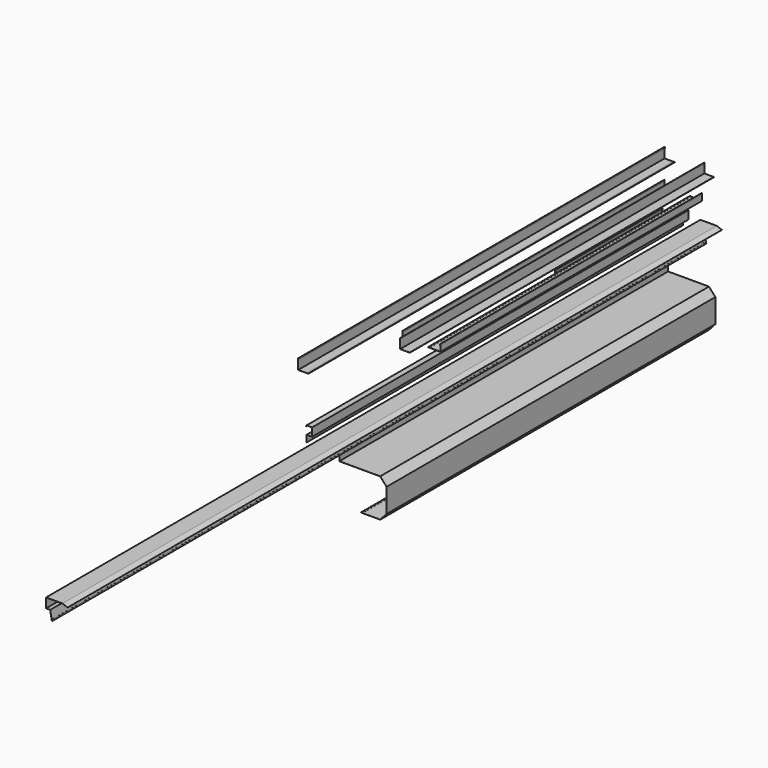
from build123d import *

# Parameters (mm, degrees)
F1_DEPTH  = 3360
F3_DEPTH  = 2790
F5_DEPTH  = 2400
F7_DEPTH  = 2400
F9_DEPTH  = 980
F11_DEPTH = 3450
F13_DEPTH = 6000
F15_DEPTH = 3015


# Not quite as in the source:
# - ends of sketch curves that miss each other by under 0.0002 mm in the source are joined


with BuildPart() as f1:
    # F0 (on Front) → F1 (new body)
    with BuildSketch(Plane.XZ):
        with BuildLine():
            Line((0, -75), (0, -0.5))
            ThreePointArc((0, -0.5), (0.1464466094, -0.1464466094), (0.5, 0))
            ThreePointArc((0.5, 0), (0.8535533906, -0.1464466094), (1, -0.5))
            Line((1, -0.5), (1, -10))
            Line((1, -10), (1.5, -10))
            Line((1.5, -10), (1.5, -0.5))
            ThreePointArc((1.5, -0.5), (1.2071067812, 0.2071067812), (0.5, 0.5))
            ThreePointArc((0.5, 0.5), (-0.2071067812, 0.2071067812), (-0.5, -0.5))
            Line((-0.5, -0.5), (-0.5, -75.5))
            Line((-0.5, -75.5), (74.5, -75.5))
            ThreePointArc((74.5, -75.5), (75.2071067812, -75.2071067812), (75.5, -74.5))
            ThreePointArc((75.5, -74.5), (75.2071067812, -73.7928932188), (74.5, -73.5))
            Line((74.5, -73.5), (65, -73.5))
            Line((65, -73.5), (65, -74))
            Line((65, -74), (74.5, -74))
            ThreePointArc((74.5, -74), (74.8535533906, -74.1464466094), (75, -74.5))
            ThreePointArc((75, -74.5), (74.8535533906, -74.8535533906), (74.5, -75))
            Line((74.5, -75), (0, -75))
        make_face()
    extrude(amount=F1_DEPTH)


with BuildPart() as f3:
    # F2 (on Front) → F3 (new body)
    with BuildSketch(Plane.XZ):
        with BuildLine():
            Line((291.6689515114, -7.9969086051), (291.6689515114, -77.4969086051))
            Line((291.6689515114, -77.4969086051), (361.1689515114, -77.4969086051))
            ThreePointArc((361.1689515114, -77.4969086051), (361.522504902, -77.6433552145), (361.6689515114, -77.9969086051))
            ThreePointArc((361.6689515114, -77.9969086051), (361.522504902, -78.3504619957), (361.1689515114, -78.4969086051))
            Line((361.1689515114, -78.4969086051), (351.6689515114, -78.4969086051))
            Line((351.6689515114, -78.4969086051), (351.6689515114, -78.9969086051))
            Line((351.6689515114, -78.9969086051), (361.1689515114, -78.9969086051))
            ThreePointArc((361.1689515114, -78.9969086051), (361.8760582926, -78.7040153863), (362.1689515114, -77.9969086051))
            ThreePointArc((362.1689515114, -77.9969086051), (361.8760582926, -77.2898018239), (361.1689515114, -76.9969086051))
            Line((361.1689515114, -76.9969086051), (292.1689515114, -76.9969086051))
            Line((292.1689515114, -76.9969086051), (292.1689515114, -7.9969086051))
            ThreePointArc((292.1689515114, -7.9969086051), (291.8760582926, -7.2898018239), (291.1689515114, -6.9969086051))
            ThreePointArc((291.1689515114, -6.9969086051), (290.4618447302, -7.2898018239), (290.1689515114, -7.9969086051))
            Line((290.1689515114, -7.9969086051), (290.1689515114, -17.4969086051))
            Line((290.1689515114, -17.4969086051), (290.6689515114, -17.4969086051))
            Line((290.6689515114, -17.4969086051), (290.6689515114, -7.9969086051))
            ThreePointArc((290.6689515114, -7.9969086051), (290.8153981208, -7.6433552145), (291.1689515114, -7.4969086051))
            ThreePointArc((291.1689515114, -7.4969086051), (291.522504902, -7.6433552145), (291.6689515114, -7.9969086051))
        make_face()
    extrude(amount=F3_DEPTH)


with BuildPart() as f5:
    # F4 (on Front) → F5 (new body)
    with BuildSketch(Plane.XZ):
        with BuildLine():
            Line((0, -212.6881961823), (0, -222.1881961823))
            Line((0, -222.1881961823), (0.5, -222.1881961823))
            Line((0.5, -222.1881961823), (0.5, -212.6881961823))
            ThreePointArc((0.5, -212.6881961823), (0.2071067812, -211.9810894011), (-0.5, -211.6881961823))
            ThreePointArc((-0.5, -211.6881961823), (-1.2071067812, -211.9810894011), (-1.5, -212.6881961823))
            Line((-1.5, -212.6881961823), (-1.5, -262.6881961823))
            Line((-1.5, -262.6881961823), (99.5, -262.6881961823))
            Line((99.5, -262.6881961823), (99.5, -212.6881961823))
            ThreePointArc((99.5, -212.6881961823), (99.2071067812, -211.9810894011), (98.5, -211.6881961823))
            ThreePointArc((98.5, -211.6881961823), (97.7928932188, -211.9810894011), (97.5, -212.6881961823))
            Line((97.5, -212.6881961823), (97.5, -222.1881961823))
            Line((97.5, -222.1881961823), (98, -222.1881961823))
            Line((98, -222.1881961823), (98, -212.6881961823))
            ThreePointArc((98, -212.6881961823), (98.1464466094, -212.3346427917), (98.5, -212.1881961823))
            ThreePointArc((98.5, -212.1881961823), (98.8535533906, -212.3346427917), (99, -212.6881961823))
            Line((99, -212.6881961823), (99, -262.1881961823))
            Line((99, -262.1881961823), (-1, -262.1881961823))
            Line((-1, -262.1881961823), (-1, -212.6881961823))
            ThreePointArc((-1, -212.6881961823), (-0.8535533906, -212.3346427917), (-0.5, -212.1881961823))
            ThreePointArc((-0.5, -212.1881961823), (-0.1464466094, -212.3346427917), (0, -212.6881961823))
        make_face()
    extrude(amount=F5_DEPTH)


with BuildPart() as f7:
    # F6 (on Front) → F7 (new body)
    with BuildSketch(Plane.XZ):
        with BuildLine():
            Line((186.1295764446, -256.9942643642), (195.6295764446, -256.9942643642))
            Line((195.6295764446, -256.9942643642), (195.6295764446, -256.4942643642))
            Line((195.6295764446, -256.4942643642), (186.1295764446, -256.4942643642))
            ThreePointArc((186.1295764446, -256.4942643642), (185.4224696634, -256.7871575831), (185.1295764446, -257.4942643642))
            ThreePointArc((185.1295764446, -257.4942643642), (185.4224696634, -258.2013711454), (186.1295764446, -258.4942643642))
            Line((186.1295764446, -258.4942643642), (276.1295764446, -258.4942643642))
            Line((276.1295764446, -258.4942643642), (276.1295764446, -208.4942643642))
            ThreePointArc((276.1295764446, -208.4942643642), (275.8366832258, -207.7871575831), (275.1295764446, -207.4942643642))
            ThreePointArc((275.1295764446, -207.4942643642), (274.4224696634, -207.7871575831), (274.1295764446, -208.4942643642))
            Line((274.1295764446, -208.4942643642), (274.1295764446, -217.9942643642))
            Line((274.1295764446, -217.9942643642), (274.6295764446, -217.9942643642))
            Line((274.6295764446, -217.9942643642), (274.6295764446, -208.4942643642))
            ThreePointArc((274.6295764446, -208.4942643642), (274.776023054, -208.1407109736), (275.1295764446, -207.9942643642))
            ThreePointArc((275.1295764446, -207.9942643642), (275.4831298352, -208.1407109736), (275.6295764446, -208.4942643642))
            Line((275.6295764446, -208.4942643642), (275.6295764446, -257.9942643642))
            Line((275.6295764446, -257.9942643642), (186.1295764446, -257.9942643642))
            ThreePointArc((186.1295764446, -257.9942643642), (185.776023054, -257.8478177548), (185.6295764446, -257.4942643642))
            ThreePointArc((185.6295764446, -257.4942643642), (185.776023054, -257.1407109736), (186.1295764446, -256.9942643642))
        make_face()
    extrude(amount=F7_DEPTH)


with BuildPart() as f9:
    # F8 (on Front) → F9 (new body)
    with BuildSketch(Plane.XZ):
        with BuildLine():
            Line((-18.0000039637, -452.1825845242), (-18.0000039637, -402.6825845242))
            ThreePointArc((-18.0000039637, -402.6825845242), (-17.8535573543, -402.3290311336), (-17.5000039637, -402.1825845242))
            ThreePointArc((-17.5000039637, -402.1825845242), (-17.1464505731, -402.3290311336), (-17.0000039637, -402.6825845242))
            Line((-17.0000039637, -402.6825845242), (-17.0000039637, -412.1825845242))
            Line((-17.0000039637, -412.1825845242), (-16.5000039637, -412.1825845242))
            Line((-16.5000039637, -412.1825845242), (-16.5000039637, -402.6825845242))
            ThreePointArc((-16.5000039637, -402.6825845242), (-16.7928971825, -401.975477743), (-17.5000039637, -401.6825845242))
            ThreePointArc((-17.5000039637, -401.6825845242), (-18.2071107449, -401.975477743), (-18.5000039637, -402.6825845242))
            Line((-18.5000039637, -402.6825845242), (-18.5000039637, -452.6825845242))
            Line((-18.5000039637, -452.6825845242), (56.4999960363, -452.6825845242))
            ThreePointArc((56.4999960363, -452.6825845242), (57.2071028175, -452.3896913053), (57.4999960363, -451.6825845242))
            ThreePointArc((57.4999960363, -451.6825845242), (57.2071028175, -450.975477743), (56.4999960363, -450.6825845242))
            Line((56.4999960363, -450.6825845242), (46.9999960363, -450.6825845242))
            Line((46.9999960363, -450.6825845242), (46.9999960363, -451.1825845242))
            Line((46.9999960363, -451.1825845242), (56.4999960363, -451.1825845242))
            ThreePointArc((56.4999960363, -451.1825845242), (56.8535494269, -451.3290311336), (56.9999960363, -451.6825845242))
            ThreePointArc((56.9999960363, -451.6825845242), (56.8535494269, -452.0361379147), (56.4999960363, -452.1825845242))
            Line((56.4999960363, -452.1825845242), (-18.0000039637, -452.1825845242))
        make_face()
    extrude(amount=F9_DEPTH)


with BuildPart() as f11:
    # F10 (on Front) → F11 (new body)
    with BuildSketch(Plane.XZ):
        with BuildLine():
            Line((128.682345044, -362.0913009151), (133.682345044, -353.4310468772))
            Line((133.682345044, -353.4310468772), (173.682345044, -353.4310468772))
            Line((173.682345044, -353.4310468772), (173.682345044, -413.4310468772))
            Line((173.682345044, -413.4310468772), (133.682345044, -413.4310468772))
            Line((133.682345044, -413.4310468772), (133.682345044, -462.9310468772))
            ThreePointArc((133.682345044, -462.9310468772), (133.5358984346, -463.2846002678), (133.182345044, -463.4310468772))
            ThreePointArc((133.182345044, -463.4310468772), (132.8287916534, -463.2846002678), (132.682345044, -462.9310468772))
            Line((132.682345044, -462.9310468772), (132.682345044, -453.4310468772))
            Line((132.682345044, -453.4310468772), (132.182345044, -453.4310468772))
            Line((132.182345044, -453.4310468772), (132.182345044, -462.9310468772))
            ThreePointArc((132.182345044, -462.9310468772), (132.4752382628, -463.6381536584), (133.182345044, -463.9310468772))
            ThreePointArc((133.182345044, -463.9310468772), (133.8894518252, -463.6381536584), (134.182345044, -462.9310468772))
            Line((134.182345044, -462.9310468772), (134.182345044, -413.9310468772))
            Line((134.182345044, -413.9310468772), (174.182345044, -413.9310468772))
            Line((174.182345044, -413.9310468772), (174.182345044, -352.9310468772))
            Line((174.182345044, -352.9310468772), (133.3936699094, -352.9310468772))
            Line((133.3936699094, -352.9310468772), (128.2493323421, -361.8413009151))
            Line((128.2493323421, -361.8413009151), (128.682345044, -362.0913009151))
        make_face()
    extrude(amount=F11_DEPTH)


with BuildPart() as f13:
    # F12 (on Front) → F13 (new body)
    with BuildSketch(Plane.XZ):
        with BuildLine():
            Line((262.9618349219, -386.152170803), (382.9618349219, -386.152170803))
            Line((382.9618349219, -386.152170803), (420.5495397534, -399.8329765361))
            Line((420.5495397534, -399.8329765361), (420.720549825, -399.3631302257))
            Line((420.720549825, -399.3631302257), (383.0499984123, -385.652170803))
            Line((383.0499984123, -385.652170803), (262.4618349219, -385.652170803))
            Line((262.4618349219, -385.652170803), (262.4618349219, -456.652170803))
            Line((262.4618349219, -456.652170803), (292.5422851063, -456.652170803))
            Line((292.5422851063, -456.652170803), (304.5379793933, -524.6831337262))
            ThreePointArc((304.5379793933, -524.6831337262), (304.9492107099, -525.3286375928), (305.696435324, -525.4942933016))
            ThreePointArc((305.696435324, -525.4942933016), (306.3419391906, -525.0830619849), (306.5075948993, -524.3358373709))
            Line((306.5075948993, -524.3358373709), (304.8579372115, -514.9801637173))
            Line((304.8579372115, -514.9801637173), (304.365533335, -515.0669878061))
            Line((304.365533335, -515.0669878061), (306.0151910228, -524.4226614597))
            ThreePointArc((306.0151910228, -524.4226614597), (305.9323631684, -524.7962737667), (305.6096112351, -525.001889425))
            ThreePointArc((305.6096112351, -525.001889425), (305.2359989281, -524.9190615707), (305.0303832698, -524.5963096374))
            Line((305.0303832698, -524.5963096374), (292.9618349219, -456.152170803))
            Line((292.9618349219, -456.152170803), (262.9618349219, -456.152170803))
            Line((262.9618349219, -456.152170803), (262.9618349219, -386.152170803))
        make_face()
    extrude(amount=F13_DEPTH)


with BuildPart() as f15:
    # F14 (on Front) → F15 (new body)
    with BuildSketch(Plane.XZ):
        with BuildLine():
            ThreePointArc((24.8575090319, -757.0222418248), (25.2110624225, -757.1686884342), (25.3575090319, -757.5222418248))
            Line((25.3575090319, -757.5222418248), (25.3575090319, -797.0222418248))
            Line((25.3575090319, -797.0222418248), (325.3575090319, -797.0222418248))
            Line((325.3575090319, -797.0222418248), (372.196651477, -849.0423796082))
            Line((372.196651477, -849.0423796082), (372.196651477, -1024.0423796082))
            Line((372.196651477, -1024.0423796082), (325.3575090319, -1076.0625173916))
            Line((325.3575090319, -1076.0625173916), (185.8575090319, -1076.0625173916))
            ThreePointArc((185.8575090319, -1076.0625173916), (185.5039556413, -1075.9160707822), (185.3575090319, -1075.5625173916))
            ThreePointArc((185.3575090319, -1075.5625173916), (185.5039556413, -1075.2089640011), (185.8575090319, -1075.0625173916))
            Line((185.8575090319, -1075.0625173916), (195.3575090319, -1075.0625173916))
            Line((195.3575090319, -1075.0625173916), (195.3575090319, -1074.5625173916))
            Line((195.3575090319, -1074.5625173916), (185.8575090319, -1074.5625173916))
            ThreePointArc((185.8575090319, -1074.5625173916), (184.857509032, -1075.5625325785), (185.8575090319, -1076.5625173916))
            Line((185.8575090319, -1076.5625173916), (325.5801233745, -1076.5625173916))
            Line((325.5801233745, -1076.5625173916), (372.696651477, -1024.2343116257))
            Line((372.696651477, -1024.2343116257), (372.696651477, -848.8504475907))
            Line((372.696651477, -848.8504475907), (325.5801233745, -796.5222418248))
            Line((325.5801233745, -796.5222418248), (25.8575090319, -796.5222418248))
            Line((25.8575090319, -796.5222418248), (25.8575090319, -757.5222418248))
            ThreePointArc((25.8575090319, -757.5222418248), (25.5646158131, -756.8151350436), (24.8575090319, -756.5222418248))
            ThreePointArc((24.8575090319, -756.5222418248), (24.1504022507, -756.8151350436), (23.8575090319, -757.5222418248))
            Line((23.8575090319, -757.5222418248), (23.8575090319, -767.0222418248))
            Line((23.8575090319, -767.0222418248), (24.3575090319, -767.0222418248))
            Line((24.3575090319, -767.0222418248), (24.3575090319, -757.5222418248))
            ThreePointArc((24.3575090319, -757.5222418248), (24.5039556413, -757.1686884342), (24.8575090319, -757.0222418248))
        make_face()
    extrude(amount=F15_DEPTH)


solid = Compound([f1.part, f3.part, f5.part, f7.part, f9.part, f11.part, f13.part, f15.part])
